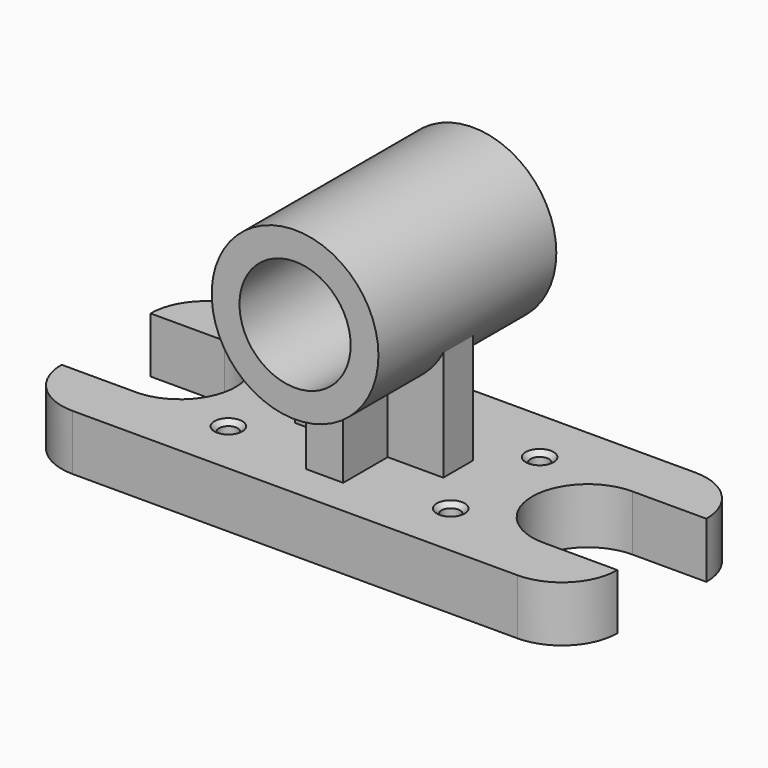
from build123d import *

# Parameters (mm, degrees)
F0_W            = 762
F0_H            = 304.8
F1_DEPTH        = 76.2
F3_DEPTH        = 203.2
F4_R            = 114.3
F4_R_2          = 76.2
F5_DEPTH        = 152.4
F6_DEPTH        = 152.4
F8_R            = 76.2
F10_DEPTH       = 76.201
F11_D           = 25.4
F11_CSINK_D     = 38.1
F11_CSINK_ANGLE = 90


# Not quite as in the source:
# - a pattern or mirror of a feature is missing from the dataset's text; its kind, count and spacing are read off the source's solid


with BuildPart() as f1:
    # F0 (on Top) → F1 (new body)
    with BuildSketch(Plane.XY):
        Rectangle(F0_W, F0_H)
    extrude(amount=F1_DEPTH)

    # F2 (on face) → F3 (join)
    with BuildSketch(Plane.XY.offset(76.2)):
        Polygon((101.6, -25.4), (101.6, 25.4), (25.4, 25.4), (25.4, 101.6), (-25.4, 101.6), (-25.4, 25.4), (-101.6, 25.4), (-101.6, -25.4), (-25.4, -25.4), (-25.4, -101.6), (25.4, -101.6), (25.4, -25.4), align=None)
    extrude(amount=F3_DEPTH)

    # F4 (on Front) → F5 (join, symmetric)
    with BuildSketch(Plane.XZ):
        with Locations((0, 279.4)):
            Circle(F4_R)
        with Locations((0, 279.4)):
            Circle(F4_R_2, mode=Mode.SUBTRACT)
    extrude(amount=F5_DEPTH, both=True)

    # F4 (on Front) → F6 (cut, symmetric)
    with BuildSketch(Plane.XZ):
        with Locations((0, 279.4)):
            Circle(F4_R_2)
    extrude(amount=F6_DEPTH, both=True, mode=Mode.SUBTRACT)

    # F8
    f8_edges = [f1.edges().sort_by_distance(p)[0] for p in [
        (381, 152.4, 38.1),
        (-381, 152.4, 38.1),
        (381, -152.4, 38.1),
        (-381, -152.4, 38.1),
    ]]
    fillet(f8_edges, radius=F8_R)

    # F9 (on face) → F10 (cut, through all)
    with BuildSketch(Plane.XY.offset(76.2)):
        with BuildLine():
            Line((-381, -76.2), (-279.4, -76.2))
            ThreePointArc((-279.4, -76.2), (-203.2, 0), (-279.4, 76.2))
            Line((-279.4, 76.2), (-381, 76.2))
            Line((-381, 76.2), (-381, -76.2))
        make_face()
    f10 = extrude(amount=-F10_DEPTH, mode=Mode.SUBTRACT)

    # F10_copies: F10 across plane
    add(f10.mirror(Plane(origin=(0, 0, 0), x_dir=(0, 0, 1), z_dir=(1, 0, 0))), mode=Mode.SUBTRACT)

    # F11 (through all)
    with Locations(Plane.XY.offset(76.2)):
        with Locations((-152.4, 76.2)):
            f11 = CounterSinkHole(F11_D / 2, F11_CSINK_D / 2, counter_sink_angle=F11_CSINK_ANGLE)

    # F11_copies: F11 across plane
    add(f11.mirror(Plane(origin=(0, 0, 0), x_dir=(0, 0, -1), z_dir=(0, -1, 0))), mode=Mode.SUBTRACT)

    # F11_copies1: F11 across plane
    add(f11.mirror(Plane(origin=(0, 0, 0), x_dir=(0, 0, 1), z_dir=(1, 0, 0))), mode=Mode.SUBTRACT)

    # F11_copies2: F11 across plane
    add(f11.mirror(Plane(origin=(0, 0, 0), x_dir=(0.4472135955, 0.894427191, 0), z_dir=(0.894427191, -0.4472135955, 0))), mode=Mode.SUBTRACT)


solid = f1.part
